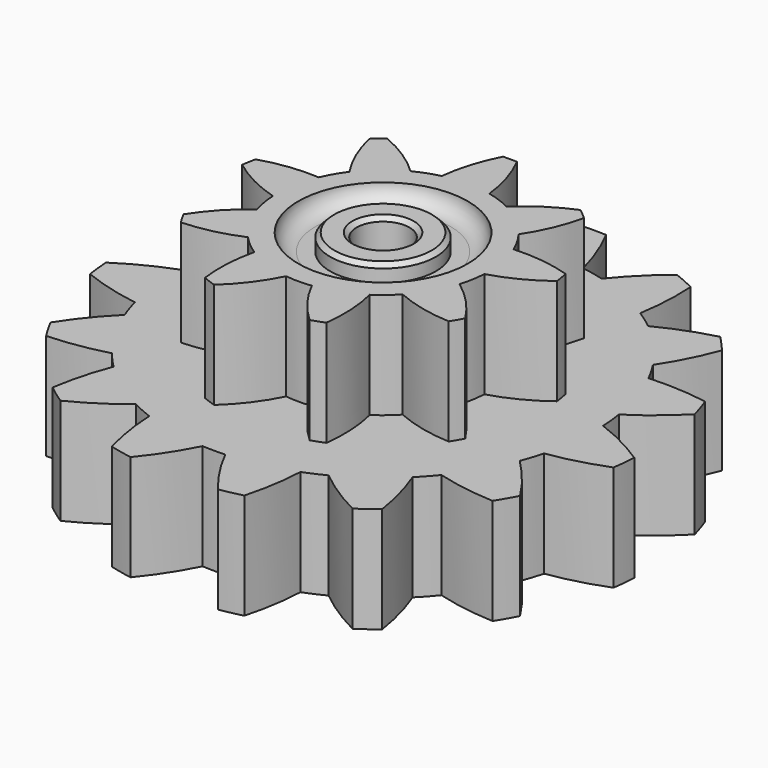
from build123d import *

# Parameters (mm, degrees)
F0_R     = 4.7625
F0_R_2   = 1.5875
F1_DEPTH = 6.35
F2_COUNT = 15
F3_R     = 4.7625
F3_R_2   = 3.175
F3_R_3   = 1.5875
F4_DEPTH = 6.35
F5_R     = 5.08
F5_R_2   = 3.175
F6_DEPTH = 1.016
F7_R     = 1.01599
F8_SIZE  = 0.254


# Not quite as in the source:
# - a fillet or chamfer is up to 0.001 mm smaller than in the source, because OpenCascade refuses the exact size


with BuildPart() as f1:
    # F0 (on Top) → F1 (new body)
    with BuildSketch(Plane.XY):
        with BuildLine():
            ThreePointArc((-1.9696004156, 12.5463410683), (-8.2545767524, -9.6515264409), (12.7, 0))
            ThreePointArc((12.7, 0), (9.6515264409, 8.2545767524), (1.9696004156, 12.5463410683))
            ThreePointArc((1.9696004156, 12.5463410683), (0, 12.7), (-1.9696004156, 12.5463410683))
        make_face()
        Circle(F0_R, mode=Mode.SUBTRACT)
        with BuildLine():
            ThreePointArc((-1.9696004156, 12.5463410683), (0, 12.7), (1.9696004156, 12.5463410683))
            ThreePointArc((1.9696004156, 12.5463410683), (1.4239736696, 14.2389394562), (0.6924577744, 15.8598905176))
            ThreePointArc((0.6924577744, 15.8598905176), (0, 15.875), (-0.6924577744, 15.8598905176))
            ThreePointArc((-0.6924577744, 15.8598905176), (-1.4239736696, 14.2389394562), (-1.9696004156, 12.5463410683))
        make_face()
        Circle(F0_R)
        Circle(F0_R_2, mode=Mode.SUBTRACT)
    extrude(amount=F1_DEPTH)

    # F2: F1 ×15 about axis
    f2_axis = Axis((0, 0, 0), (0, 0, -1))


with BuildPart() as f1_1:
    add(f1.part)
    for i in range(1, F2_COUNT):
        add(f1.part.rotate(f2_axis, i * 360 / F2_COUNT))

    # F3 (on face) → F4 (join)
    with BuildSketch(Plane.XY.offset(6.35)):
        with BuildLine():
            ThreePointArc((6.3411298165, -0.3355184801), (6.3477820668, -0.1678178556), (6.35, 0))
            ThreePointArc((6.35, 0), (6.222203729, 1.2675491134), (5.8439588173, 2.4840783686))
            ThreePointArc((5.8439588173, 2.4840783686), (5.499261314, 3.175), (5.0732543809, 3.8189776102))
            ThreePointArc((5.0732543809, 3.8189776102), (4.0817013215, 4.8643822138), (2.879997381, 5.6593387498))
            ThreePointArc((2.879997381, 5.6593387498), (2.1718279101, 5.967048142), (1.4315468375, 6.1865316335))
            ThreePointArc((1.4315468375, 6.1865316335), (0, 6.35), (-1.4315468375, 6.1865316335))
            ThreePointArc((-1.4315468375, 6.1865316335), (-2.1718279101, 5.967048142), (-2.879997381, 5.6593387498))
            ThreePointArc((-2.879997381, 5.6593387498), (-4.0817013215, 4.8643822138), (-5.0732543809, 3.8189776102))
            ThreePointArc((-5.0732543809, 3.8189776102), (-5.499261314, 3.175), (-5.8439588173, 2.4840783686))
            ThreePointArc((-5.8439588173, 2.4840783686), (-6.2535292316, 1.1026659282), (-6.3411298165, -0.3355184801))
            ThreePointArc((-6.3411298165, -0.3355184801), (-6.2535292316, -1.1026659282), (-6.0734669747, -1.8535098888))
            ThreePointArc((-6.0734669747, -1.8535098888), (-5.499261314, -3.175), (-4.6419201372, -4.3330217447))
            ThreePointArc((-4.6419201372, -4.3330217447), (-4.0817013215, -4.8643822138), (-3.4611324355, -5.3238202697))
            ThreePointArc((-3.4611324355, -5.3238202697), (-2.1718279101, -5.967048142), (-0.7707044365, -6.3030559788))
            ThreePointArc((-0.7707044365, -6.3030559788), (0, -6.35), (0.7707044365, -6.3030559788))
            ThreePointArc((0.7707044365, -6.3030559788), (2.1718279101, -5.967048142), (3.4611324355, -5.3238202697))
            ThreePointArc((3.4611324355, -5.3238202697), (4.0817013215, -4.8643822138), (4.6419201372, -4.3330217447))
            ThreePointArc((4.6419201372, -4.3330217447), (5.499261314, -3.175), (6.0734669747, -1.8535098888))
            ThreePointArc((6.0734669747, -1.8535098888), (6.2535292316, -1.1026659282), (6.3411298165, -0.3355184801))
        make_face()
        Circle(F3_R, mode=Mode.SUBTRACT)
        with BuildLine():
            ThreePointArc((5.8439588173, 2.4840783686), (6.222203729, 1.2675491134), (6.35, 0))
            ThreePointArc((6.35, 0), (6.3477820668, -0.1678178556), (6.3411298165, -0.3355184801))
            ThreePointArc((6.3411298165, -0.3355184801), (7.9650557648, 0.3109444224), (9.4435123046, 1.2432619809))
            ThreePointArc((9.4435123046, 1.2432619809), (9.3802938474, 1.6539988923), (9.2992194678, 2.0615873228))
            ThreePointArc((9.2992194678, 2.0615873228), (7.5910533822, 2.4320173351), (5.8439588173, 2.4840783686))
        make_face()
        with BuildLine():
            ThreePointArc((2.879997381, 5.6593387498), (4.0817013215, 4.8643822138), (5.0732543809, 3.8189776102))
            ThreePointArc((5.0732543809, 3.8189776102), (5.9017154857, 5.358036403), (6.4349967275, 7.0225666331))
            ThreePointArc((6.4349967275, 7.0225666331), (6.1225519823, 7.2965733207), (5.7984526113, 7.5566905663))
            ThreePointArc((5.7984526113, 7.5566905663), (4.2518136514, 6.7424684237), (2.879997381, 5.6593387498))
        make_face()
        with BuildLine():
            ThreePointArc((8.448778186, -4.3981555411), (7.3783548704, -3.0164016935), (6.0734669747, -1.8535098888))
            ThreePointArc((6.0734669747, -1.8535098888), (5.499261314, -3.175), (4.6419201372, -4.3330217447))
            ThreePointArc((4.6419201372, -4.3330217447), (6.3014579298, -4.8816419092), (8.0333035214, -5.1177787695))
            ThreePointArc((8.0333035214, -5.1177787695), (8.248891971, -4.7625), (8.448778186, -4.3981555411))
        make_face()
        with BuildLine():
            ThreePointArc((-1.4315468375, 6.1865316335), (0, 6.35), (1.4315468375, 6.1865316335))
            ThreePointArc((1.4315468375, 6.1865316335), (1.0768969406, 7.8980436026), (0.4154746647, 9.5159343106))
            ThreePointArc((0.4154746647, 9.5159343106), (0, 9.525), (-0.4154746647, 9.5159343106))
            ThreePointArc((-0.4154746647, 9.5159343106), (-1.0768969406, 7.8980436026), (-1.4315468375, 6.1865316335))
        make_face()
        with BuildLine():
            ThreePointArc((3.6450596933, -8.7999525472), (3.7132421134, -7.0534128461), (3.4611324355, -5.3238202697))
            ThreePointArc((3.4611324355, -5.3238202697), (2.1718279101, -5.967048142), (0.7707044365, -6.3030559788))
            ThreePointArc((0.7707044365, -6.3030559788), (1.6893378965, -7.790053738), (2.8642227403, -9.0841539559))
            ThreePointArc((2.8642227403, -9.0841539559), (3.2577418652, -8.950572213), (3.6450596933, -8.7999525472))
        make_face()
        with BuildLine():
            ThreePointArc((-5.0732543809, 3.8189776102), (-4.0817013215, 4.8643822138), (-2.879997381, 5.6593387498))
            ThreePointArc((-2.879997381, 5.6593387498), (-4.2518136514, 6.7424684237), (-5.7984526113, 7.5566905663))
            ThreePointArc((-5.7984526113, 7.5566905663), (-6.1225519823, 7.2965733207), (-6.4349967275, 7.0225666331))
            ThreePointArc((-6.4349967275, 7.0225666331), (-5.9017154857, 5.358036403), (-5.0732543809, 3.8189776102))
        make_face()
        with BuildLine():
            ThreePointArc((-2.8642227403, -9.0841539559), (-1.6893378965, -7.790053738), (-0.7707044365, -6.3030559788))
            ThreePointArc((-0.7707044365, -6.3030559788), (-2.1718279101, -5.967048142), (-3.4611324355, -5.3238202697))
            ThreePointArc((-3.4611324355, -5.3238202697), (-3.7132421134, -7.0534128461), (-3.6450596933, -8.7999525472))
            ThreePointArc((-3.6450596933, -8.7999525472), (-3.2577418652, -8.950572213), (-2.8642227403, -9.0841539559))
        make_face()
        with BuildLine():
            ThreePointArc((-6.3411298165, -0.3355184801), (-6.2535292316, 1.1026659282), (-5.8439588173, 2.4840783686))
            ThreePointArc((-5.8439588173, 2.4840783686), (-7.5910533822, 2.4320173351), (-9.2992194678, 2.0615873228))
            ThreePointArc((-9.2992194678, 2.0615873228), (-9.3802938474, 1.6539988923), (-9.4435123046, 1.2432619809))
            ThreePointArc((-9.4435123046, 1.2432619809), (-7.9650557648, 0.3109444224), (-6.3411298165, -0.3355184801))
        make_face()
        with BuildLine():
            ThreePointArc((-8.0333035214, -5.1177787695), (-6.3014579298, -4.8816419092), (-4.6419201372, -4.3330217447))
            ThreePointArc((-4.6419201372, -4.3330217447), (-5.499261314, -3.175), (-6.0734669747, -1.8535098888))
            ThreePointArc((-6.0734669747, -1.8535098888), (-7.3783548704, -3.0164016935), (-8.448778186, -4.3981555411))
            ThreePointArc((-8.448778186, -4.3981555411), (-8.248891971, -4.7625), (-8.0333035214, -5.1177787695))
        make_face()
        Circle(F3_R)
        Circle(F3_R_2, mode=Mode.SUBTRACT)
        Circle(F3_R_2)
        Circle(F3_R_3, mode=Mode.SUBTRACT)
    extrude(amount=F4_DEPTH)

    # F5 (on face) → F6 (cut)
    with BuildSketch(Plane.XY.offset(12.7)):
        Circle(F5_R)
        Circle(F5_R_2, mode=Mode.SUBTRACT)
    extrude(amount=-F6_DEPTH, mode=Mode.SUBTRACT)

    # F7 (radius 1.016 in the source; OpenCascade refuses exactly that, so slightly less here)
    f7_edges = [f1_1.edges().sort_by_distance(p)[0] for p in [
        (-5.08, 0, 11.684),
    ]]
    fillet(f7_edges, radius=F7_R)

    # F8
    f8_edges = [f1_1.edges().sort_by_distance(p)[0] for p in [
        (-1.5875, 0, 12.7),
        (-3.175, 0, 12.7),
    ]]
    chamfer(f8_edges, length=F8_SIZE)


solid = f1_1.part
